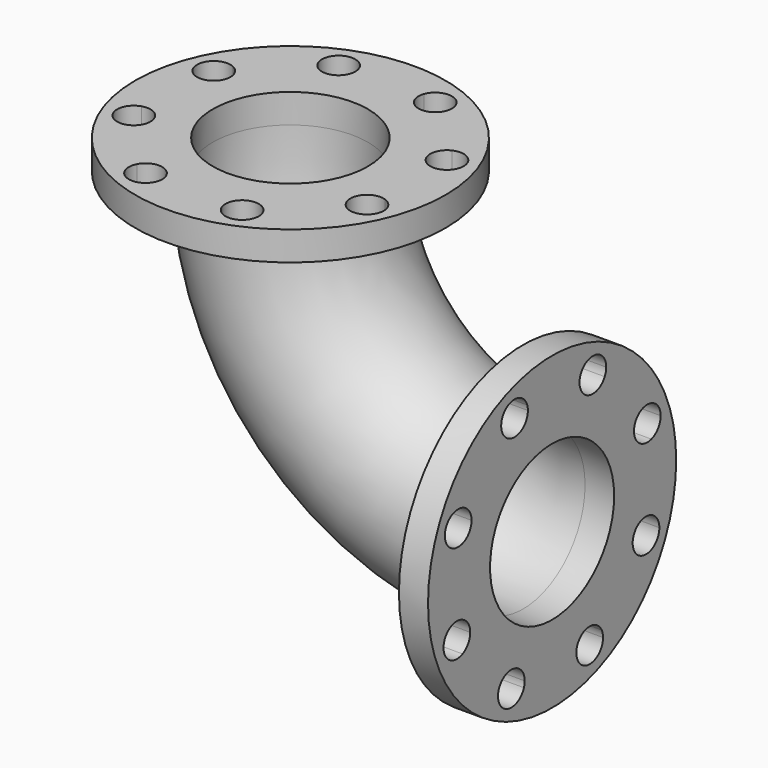
from build123d import *

# Parameters (mm, degrees)
F0_R     = 127
F0_R_2   = 76.2
F0_R_3   = 63.5
F1_DEPTH = 23.8125
F2_ANGLE = 90
F3_R     = 127
F3_R_2   = 76.2
F3_R_3   = 63.5
F4_DEPTH = 23.8125


with BuildPart() as f1:
    # F0 (on Top) → F1 (new body)
    with BuildSketch(Plane.XY):
        Circle(F0_R)
        with BuildLine():
            ThreePointArc((28.8603537964, 100.7217980566), (44.0561876825, 109.567966691), (55.3745369645, 96.1120001135))
            ThreePointArc((55.3745369645, 96.1120001135), (54.9915876268, 92.9004802457), (53.8642145113, 89.8690548525))
            ThreePointArc((53.8642145113, 89.8690548525), (75.3216864654, 72.8316152026), (91.628418296, 50.8137145422))
            ThreePointArc((91.628418296, 50.8137145422), (104.7703861556, 49.9996906202), (111.1174419453, 38.4632770973))
            ThreePointArc((111.1174419453, 38.4632770973), (108.4950074221, 30.41614465), (101.6347694492, 25.4592667608))
            ThreePointArc((101.6347694492, 25.4592667608), (103.9869789782, 12.8260994842), (104.775, 0))
            ThreePointArc((104.775, 0), (103.756751627, -14.5717918189), (100.7217980566, -28.8603537964))
            ThreePointArc((100.7217980565, -28.8603537964), (107.2810644551, -33.856165902), (109.7698250888, -41.7167119892))
            ThreePointArc((109.7698250888, -41.7167119892), (103.2278672199, -53.3743540483), (89.8690548525, -53.8642145113))
            ThreePointArc((89.8690548525, -53.8642145113), (72.8316152026, -75.3216864654), (50.8137145422, -91.628418296))
            ThreePointArc((50.8137145422, -91.628418296), (51.7902477967, -94.4716352042), (52.1211020726, -97.45961697))
            ThreePointArc((52.1211020726, -97.45961697), (40.5762945965, -110.9529983143), (25.4592667608, -101.6347694492))
            ThreePointArc((25.4592667608, -101.6347694492), (-1.7607462756, -104.7602042646), (-28.8603537964, -100.7217980566))
            ThreePointArc((-28.8603537964, -100.7217980566), (-47.1546461423, -108.6405696728), (-53.8642145113, -89.8690548525))
            ThreePointArc((-53.8642145113, -89.8690548525), (-75.3216864654, -72.8316152026), (-91.628418296, -50.8137145422))
            ThreePointArc((-91.628418296, -50.8137145422), (-110.1638535792, -43.4771134759), (-101.6347694492, -25.4592667608))
            ThreePointArc((-101.6347694492, -25.4592667608), (-104.7602042646, 1.7607462756), (-100.7217980566, 28.8603537964))
            ThreePointArc((-100.7217980565, 28.8603537964), (-108.6405696728, 47.1546461423), (-89.8690548525, 53.8642145113))
            ThreePointArc((-89.8690548525, 53.8642145113), (-72.8316152026, 75.3216864654), (-50.8137145422, 91.628418296))
            ThreePointArc((-50.8137145422, 91.628418296), (-43.4771134759, 110.1638535792), (-25.4592667608, 101.6347694492))
            ThreePointArc((-25.4592667608, 101.6347694492), (1.7607462756, 104.7602042646), (28.8603537964, 100.7217980566))
        make_face(mode=Mode.SUBTRACT)
        with BuildLine():
            ThreePointArc((53.8642145113, 89.8690548525), (36.278777836, 83.5834305542), (28.8603537964, 100.7217980566))
            ThreePointArc((28.8603537964, 100.7217980566), (1.7607462756, 104.7602042646), (-25.4592667608, 101.6347694492))
            ThreePointArc((-25.4592667608, 101.6347694492), (-24.969895753, 99.5726344691), (-24.805452122, 97.45961697))
            ThreePointArc((-24.805452122, 97.45961697), (-35.4752953315, 84.1326462706), (-50.8137145422, 91.628418296))
            ThreePointArc((-50.8137145422, 91.628418296), (-72.8316152026, 75.3216864654), (-89.8690548525, 53.8642145113))
            ThreePointArc((-89.8690548525, 53.8642145113), (-84.4543580543, 48.8325790955), (-82.4541751382, 41.7167119892))
            ThreePointArc((-82.4541751382, 41.7167119892), (-88.2514540263, 30.5476476476), (-100.7217980565, 28.8603537964))
            ThreePointArc((-100.7217980566, 28.8603537964), (-104.7602042646, 1.7607462756), (-101.6347694492, -25.4592667608))
            ThreePointArc((-101.6347694492, -25.4592667608), (-89.4124845227, -27.4278866452), (-83.8017919947, -38.4632770973))
            ThreePointArc((-83.8017919947, -38.4632770973), (-85.9232034471, -45.7740462829), (-91.628418296, -50.8137145422))
            ThreePointArc((-91.628418296, -50.8137145422), (-75.3216864654, -72.8316152026), (-53.8642145113, -89.8690548525))
            ThreePointArc((-53.8642145113, -89.8690548525), (-38.5051921214, -82.8371244758), (-28.0588870139, -96.1120001135))
            ThreePointArc((-28.0588870139, -96.1120001135), (-28.2607454116, -98.4514758068), (-28.8603537964, -100.7217980566))
            ThreePointArc((-28.8603537964, -100.7217980566), (-1.7607462756, -104.7602042646), (25.4592667608, -101.6347694492))
            ThreePointArc((25.4592667608, -101.6347694492), (33.4494407187, -84.7553803607), (50.8137145422, -91.628418296))
            ThreePointArc((50.8137145422, -91.628418296), (72.8316152026, -75.3216864654), (89.8690548525, -53.8642145113))
            ThreePointArc((89.8690548525, -53.8642145113), (83.5834305542, -36.278777836), (100.7217980565, -28.8603537964))
            ThreePointArc((100.7217980566, -28.8603537964), (103.756751627, -14.5717918189), (104.775, 0))
            ThreePointArc((104.775, 0), (103.9869789782, 12.8260994842), (101.6347694492, 25.4592667608))
            ThreePointArc((101.6347694492, 25.4592667608), (84.7553803607, 33.4494407187), (91.628418296, 50.8137145422))
            ThreePointArc((91.628418296, 50.8137145422), (75.3216864654, 72.8316152026), (53.8642145113, 89.8690548525))
        make_face()
        Circle(F0_R_2, mode=Mode.SUBTRACT)
        Circle(F0_R_2)
        Circle(F0_R_3, mode=Mode.SUBTRACT)
    extrude(amount=F1_DEPTH)

    # F0 (on Top) → F2 (revolve)
    with BuildSketch(Plane.XY):
        Circle(F0_R_2)
        Circle(F0_R_3, mode=Mode.SUBTRACT)
    revolve(axis=Axis((190.5, -17.9878585041, 0), (0, -1, 0)), revolution_arc=F2_ANGLE)

    # F3 (on face) → F4 (join)
    with BuildSketch(Plane.YZ.offset(190.5)):
        with Locations((0, -190.5)):
            Circle(F3_R)
        with BuildLine():
            ThreePointArc((28.8603537964, -89.7782019434), (44.0561876825, -80.932033309), (55.3745369645, -94.3879998865))
            ThreePointArc((55.3745369645, -94.3879998865), (54.9915876268, -97.5995197543), (53.8642145113, -100.6309451475))
            ThreePointArc((53.8642145113, -100.6309451475), (75.3216864654, -117.6683847974), (91.628418296, -139.6862854578))
            ThreePointArc((91.628418296, -139.6862854578), (104.7703861556, -140.5003093798), (111.1174419453, -152.0367229027))
            ThreePointArc((111.1174419453, -152.0367229027), (108.4950074221, -160.08385535), (101.6347694492, -165.0407332392))
            ThreePointArc((101.6347694492, -165.0407332392), (103.9869789782, -177.6739005158), (104.775, -190.5))
            ThreePointArc((104.775, -190.5), (103.756751627, -205.0717918189), (100.7217980566, -219.3603537964))
            ThreePointArc((100.7217980565, -219.3603537964), (107.2810644551, -224.356165902), (109.7698250888, -232.2167119892))
            ThreePointArc((109.7698250888, -232.2167119892), (103.2278672199, -243.8743540483), (89.8690548525, -244.3642145113))
            ThreePointArc((89.8690548525, -244.3642145113), (72.8316152026, -265.8216864654), (50.8137145422, -282.128418296))
            ThreePointArc((50.8137145422, -282.128418296), (51.7902477967, -284.9716352042), (52.1211020726, -287.95961697))
            ThreePointArc((52.1211020726, -287.95961697), (40.5762945965, -301.4529983143), (25.4592667608, -292.1347694492))
            ThreePointArc((25.4592667608, -292.1347694492), (-1.7607462756, -295.2602042646), (-28.8603537964, -291.2217980566))
            ThreePointArc((-28.8603537964, -291.2217980566), (-47.1546461423, -299.1405696728), (-53.8642145113, -280.3690548525))
            ThreePointArc((-53.8642145113, -280.3690548525), (-75.3216864654, -263.3316152026), (-91.628418296, -241.3137145422))
            ThreePointArc((-91.628418296, -241.3137145422), (-110.1638535792, -233.9771134759), (-101.6347694492, -215.9592667608))
            ThreePointArc((-101.6347694492, -215.9592667608), (-104.7602042646, -188.7392537244), (-100.7217980566, -161.6396462036))
            ThreePointArc((-100.7217980565, -161.6396462036), (-108.6405696728, -143.3453538577), (-89.8690548525, -136.6357854887))
            ThreePointArc((-89.8690548525, -136.6357854887), (-72.8316152026, -115.1783135346), (-50.8137145422, -98.871581704))
            ThreePointArc((-50.8137145422, -98.871581704), (-43.4771134759, -80.3361464208), (-25.4592667608, -88.8652305508))
            ThreePointArc((-25.4592667608, -88.8652305508), (1.7607462756, -85.7397957354), (28.8603537964, -89.7782019434))
        make_face(mode=Mode.SUBTRACT)
        with BuildLine():
            ThreePointArc((53.8642145113, -100.6309451475), (36.278777836, -106.9165694458), (28.8603537964, -89.7782019434))
            ThreePointArc((28.8603537964, -89.7782019434), (1.7607462756, -85.7397957354), (-25.4592667608, -88.8652305508))
            ThreePointArc((-25.4592667608, -88.8652305508), (-24.969895753, -90.9273655309), (-24.805452122, -93.04038303))
            ThreePointArc((-24.805452122, -93.04038303), (-35.4752953315, -106.3673537294), (-50.8137145422, -98.871581704))
            ThreePointArc((-50.8137145422, -98.871581704), (-72.8316152026, -115.1783135346), (-89.8690548525, -136.6357854887))
            ThreePointArc((-89.8690548525, -136.6357854887), (-84.4543580543, -141.6674209045), (-82.4541751382, -148.7832880108))
            ThreePointArc((-82.4541751382, -148.7832880108), (-88.2514540263, -159.9523523524), (-100.7217980565, -161.6396462036))
            ThreePointArc((-100.7217980566, -161.6396462036), (-104.7602042646, -188.7392537244), (-101.6347694492, -215.9592667608))
            ThreePointArc((-101.6347694492, -215.9592667608), (-89.4124845227, -217.9278866452), (-83.8017919947, -228.9632770973))
            ThreePointArc((-83.8017919947, -228.9632770973), (-85.9232034471, -236.2740462829), (-91.628418296, -241.3137145422))
            ThreePointArc((-91.628418296, -241.3137145422), (-75.3216864654, -263.3316152026), (-53.8642145113, -280.3690548525))
            ThreePointArc((-53.8642145113, -280.3690548525), (-38.5051921214, -273.3371244758), (-28.0588870139, -286.6120001135))
            ThreePointArc((-28.0588870139, -286.6120001135), (-28.2607454116, -288.9514758068), (-28.8603537964, -291.2217980566))
            ThreePointArc((-28.8603537964, -291.2217980566), (-1.7607462756, -295.2602042646), (25.4592667608, -292.1347694492))
            ThreePointArc((25.4592667608, -292.1347694492), (33.4494407187, -275.2553803607), (50.8137145422, -282.128418296))
            ThreePointArc((50.8137145422, -282.128418296), (72.8316152026, -265.8216864654), (89.8690548525, -244.3642145113))
            ThreePointArc((89.8690548525, -244.3642145113), (83.5834305542, -226.778777836), (100.7217980565, -219.3603537964))
            ThreePointArc((100.7217980566, -219.3603537964), (103.756751627, -205.0717918189), (104.775, -190.5))
            ThreePointArc((104.775, -190.5), (103.9869789782, -177.6739005158), (101.6347694492, -165.0407332392))
            ThreePointArc((101.6347694492, -165.0407332392), (84.7553803607, -157.0505592813), (91.628418296, -139.6862854578))
            ThreePointArc((91.628418296, -139.6862854578), (75.3216864654, -117.6683847974), (53.8642145113, -100.6309451475))
        make_face()
        with Locations((0, -190.5)):
            Circle(F3_R_2, mode=Mode.SUBTRACT)
        with Locations((0, -190.5)):
            Circle(F3_R_2)
        with Locations((0, -190.5)):
            Circle(F3_R_3, mode=Mode.SUBTRACT)
    extrude(amount=F4_DEPTH)


solid = f1.part
